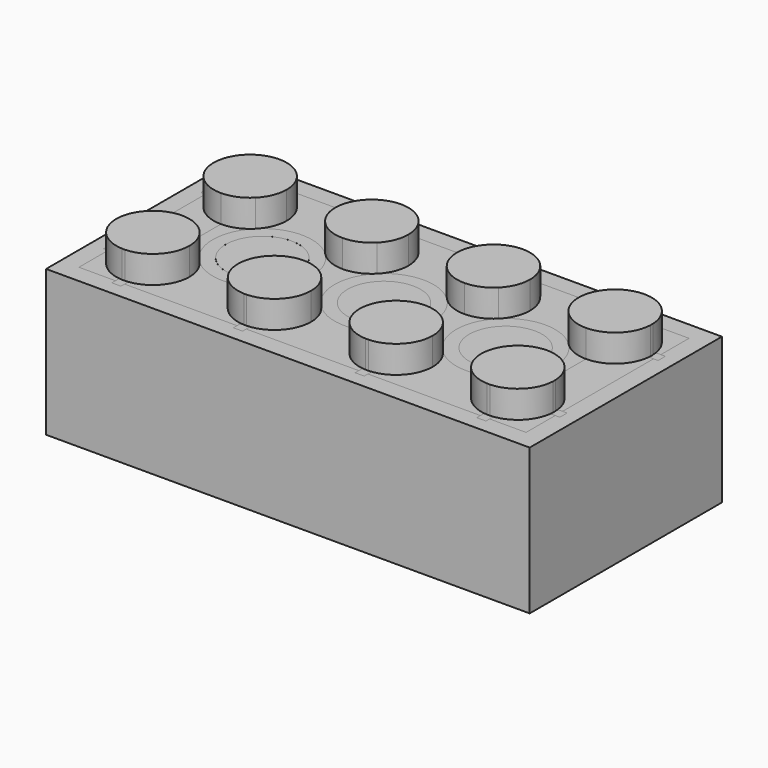
from build123d import *

# Parameters (mm, degrees)
F0_W     = 31.8
F0_H     = 15.8
F1_DEPTH = 9.6
F3_DEPTH = 1.8
F4_DEPTH = 9.6
F5_DEPTH = 1
F6_DEPTH = 1
F7_DEPTH = 1
F8_DEPTH = 1
F0_W_2   = 0.6
F0_H_2   = 0.3
F9_DEPTH = 9.6
F0_W_3   = 0.3
F0_H_3   = 0.6


# Not quite as in the source:
# - the program builds the solid bodies; features that only make, move or delete a surface that nothing else refers to are left out


with BuildPart() as f1:
    # F0 (on Top) → F1 (new body)
    with BuildSketch(Plane.XY):
        Rectangle(F0_W, F0_H)
        Polygon((-3.7, 6.7), (3.7, 6.7), (3.7, 7), (4.3, 7), (4.3, 6.7), (11.7, 6.7), (11.7, 7), (12.3, 7), (12.3, 6.7), (14.7, 6.7), (14.7, 4.3778601542), (15, 4.3778601542), (15, 3.7778601542), (14.7, 3.7778601542), (14.7, 0), (14.7, -3.7), (15, -3.7), (15, -4.3), (14.7, -4.3), (14.7, -6.7), (12.3, -6.7), (12.3, -7), (11.7, -7), (11.7, -6.7), (4.3, -6.7), (4.3, -7), (3.7, -7), (3.7, -6.7), (-3.7, -6.7), (-3.7, -7), (-4.3, -7), (-4.3, -6.7), (-11.7, -6.7), (-11.7, -7), (-12.3, -7), (-12.3, -6.7), (-14.7, -6.7), (-14.7, -4.3), (-15, -4.3), (-15, -3.7), (-14.7, -3.7), (-14.7, 0), (-14.7, 3.7), (-15, 3.7), (-15, 4.3), (-14.7, 4.3), (-14.7, 6.7), (-12.3, 6.7), (-12.3, 7), (-11.7, 7), (-11.7, 6.7), (-4.3, 6.7), (-4.3, 7), (-3.7, 7), align=None, mode=Mode.SUBTRACT)
    extrude(amount=-F1_DEPTH)


with BuildPart() as f3:
    # F0 (on Top) → F3 (new body)
    with BuildSketch(Plane.XY):
        with BuildLine():
            ThreePointArc((-14.4, 3.9056398611), (-13.6646718198, 2.2685926048), (-12, 1.5981457505))
            Line((-12, 1.5981457505), (-12, 2.7))
            ThreePointArc((-12, 2.7), (-12.9192388155, 4.9192388155), (-10.7, 4))
            Line((-10.7, 4), (-9.5981457505, 4))
            ThreePointArc((-9.5981457505, 4), (-10.2685926048, 5.6646718198), (-11.9056398611, 6.4))
            Line((-11.9056398611, 6.4), (-12.0943601389, 6.4))
            ThreePointArc((-12.0943601389, 6.4), (-13.6983674272, 5.6983674272), (-14.4, 4.0943601389))
            Line((-14.4, 4.0943601389), (-14.4, 3.9056398611))
        make_face()
        with BuildLine():
            ThreePointArc((-12, 1.5981457505), (-11.0808501792, 1.7809760157), (-10.3016325841, 2.3016325614))
            ThreePointArc((-10.3016325841, 2.3016325614), (-9.7809760219, 3.0808501643), (-9.5981457505, 4))
            Line((-9.5981457505, 4), (-10.7, 4))
            ThreePointArc((-10.7, 4), (-11.0807611845, 3.0807611845), (-12, 2.7))
            Line((-12, 2.7), (-12, 1.5981457505))
        make_face()
        with BuildLine():
            ThreePointArc((-10.7, 4), (-12.9192388155, 4.9192388155), (-12, 2.7))
            Line((-12, 2.7), (-12, 4))
            Line((-12, 4), (-10.7, 4))
        make_face()
        with BuildLine():
            Line((-12, 4), (-12, 2.7))
            ThreePointArc((-12, 2.7), (-11.0807611845, 3.0807611845), (-10.7, 4))
            Line((-10.7, 4), (-12, 4))
        make_face()
    extrude(amount=F3_DEPTH)


with BuildPart() as f3b:
    # F0 (on Top) → F3, piece 2 (new body)
    with BuildSketch(Plane.XY):
        with BuildLine():
            Line((-2.7, 4), (-1.5981457505, 4))
            ThreePointArc((-1.5981457505, 4), (-2.2685926048, 5.6646718198), (-3.9056398611, 6.4))
            Line((-3.9056398611, 6.4), (-4.0943601389, 6.4))
            ThreePointArc((-4.0943601389, 6.4), (-5.7314073952, 5.6646718198), (-6.4018542495, 4))
            Line((-6.4018542495, 4), (-5.3, 4))
            ThreePointArc((-5.3, 4), (-4, 5.3), (-2.7, 4))
        make_face()
        with BuildLine():
            ThreePointArc((-5.6983674332, 2.3016325788), (-4.9191498322, 1.7809760204), (-4, 1.5981457505))
            Line((-4, 1.5981457505), (-4, 2.7))
            ThreePointArc((-4, 2.7), (-4.9192388155, 3.0807611845), (-5.3, 4))
            Line((-5.3, 4), (-6.4018542495, 4))
            ThreePointArc((-6.4018542495, 4), (-6.2190239828, 3.0808501757), (-5.6983674332, 2.3016325788))
        make_face()
        with BuildLine():
            ThreePointArc((-4, 1.5981457505), (-3.0808501718, 1.7809760188), (-2.3016325728, 2.3016325728))
            ThreePointArc((-2.3016325728, 2.3016325728), (-1.7809760188, 3.0808501718), (-1.5981457505, 4))
            Line((-1.5981457505, 4), (-2.7, 4))
            ThreePointArc((-2.7, 4), (-3.0807611845, 3.0807611845), (-4, 2.7))
            Line((-4, 2.7), (-4, 1.5981457505))
        make_face()
        with BuildLine():
            Line((-4, 4), (-2.7, 4))
            ThreePointArc((-2.7, 4), (-4, 5.3), (-5.3, 4))
            Line((-5.3, 4), (-4, 4))
        make_face()
        with BuildLine():
            ThreePointArc((-5.3, 4), (-4.9192388155, 3.0807611845), (-4, 2.7))
            Line((-4, 2.7), (-4, 4))
            Line((-4, 4), (-5.3, 4))
        make_face()
        with BuildLine():
            Line((-4, 4), (-4, 2.7))
            ThreePointArc((-4, 2.7), (-3.0807611845, 3.0807611845), (-2.7, 4))
            Line((-2.7, 4), (-4, 4))
        make_face()
    extrude(amount=F3_DEPTH)


with BuildPart() as f3c:
    # F0 (on Top) → F3, piece 3 (new body)
    with BuildSketch(Plane.XY):
        with BuildLine():
            ThreePointArc((3.9056398611, 6.4), (2.2685926048, 5.6646718198), (1.5981457505, 4))
            Line((1.5981457505, 4), (2.7, 4))
            ThreePointArc((2.7, 4), (4, 5.3), (5.3, 4))
            Line((5.3, 4), (6.4018542495, 4))
            ThreePointArc((6.4018542495, 4), (5.7314073952, 5.6646718198), (4.0943601389, 6.4))
            Line((4.0943601389, 6.4), (3.9056398611, 6.4))
        make_face()
        with BuildLine():
            ThreePointArc((1.5981457505, 4), (1.7809760181, 3.0808501735), (2.3016325701, 2.3016325754))
            ThreePointArc((2.3016325701, 2.3016325754), (3.08085017, 1.7809760195), (4, 1.5981457505))
            Line((4, 1.5981457505), (4, 2.7))
            ThreePointArc((4, 2.7), (3.0807611845, 3.0807611845), (2.7, 4))
            Line((2.7, 4), (1.5981457505, 4))
        make_face()
        with BuildLine():
            Line((4, 2.7), (4, 1.5981457505))
            ThreePointArc((4, 1.5981457505), (4.9191498286, 1.780976019), (5.6983674279, 2.3016325734))
            ThreePointArc((5.6983674279, 2.3016325734), (6.2190239814, 3.0808501722), (6.4018542495, 4))
            Line((6.4018542495, 4), (5.3, 4))
            ThreePointArc((5.3, 4), (4.9192388155, 3.0807611845), (4, 2.7))
        make_face()
        with BuildLine():
            ThreePointArc((5.3, 4), (4, 5.3), (2.7, 4))
            Line((2.7, 4), (4, 4))
            Line((4, 4), (5.3, 4))
        make_face()
        with BuildLine():
            Line((4, 4), (2.7, 4))
            ThreePointArc((2.7, 4), (3.0807611845, 3.0807611845), (4, 2.7))
            Line((4, 2.7), (4, 4))
        make_face()
        with BuildLine():
            Line((4, 4), (4, 2.7))
            ThreePointArc((4, 2.7), (4.9192388155, 3.0807611845), (5.3, 4))
            Line((5.3, 4), (4, 4))
        make_face()
    extrude(amount=F3_DEPTH)


with BuildPart() as f3d:
    # F0 (on Top) → F3, piece 4 (new body)
    with BuildSketch(Plane.XY):
        with BuildLine():
            ThreePointArc((9.5981457505, 4), (9.7809760218, 3.0808501646), (10.3016325837, 2.3016325618))
            ThreePointArc((10.3016325837, 2.3016325618), (11.0808501789, 1.7809760159), (12, 1.5981457505))
            Line((12, 1.5981457505), (12, 2.7))
            ThreePointArc((12, 2.7), (11.0807611845, 3.0807611845), (10.7, 4))
            Line((10.7, 4), (9.5981457505, 4))
        make_face()
        with BuildLine():
            ThreePointArc((11.9056398611, 6.4), (10.2685926048, 5.6646718198), (9.5981457505, 4))
            Line((9.5981457505, 4), (10.7, 4))
            ThreePointArc((10.7, 4), (12, 5.3), (13.3, 4))
            ThreePointArc((13.3, 4), (12.9192388155, 3.0807611845), (12, 2.7))
            Line((12, 2.7), (12, 1.5981457505))
            ThreePointArc((12, 1.5981457505), (13.6646718198, 2.2685926048), (14.4, 3.9056398611))
            Line((14.4, 3.9056398611), (14.4, 4.0943601389))
            ThreePointArc((14.4, 4.0943601389), (13.6983674272, 5.6983674272), (12.0943601389, 6.4))
            Line((12.0943601389, 6.4), (11.9056398611, 6.4))
        make_face()
        with BuildLine():
            ThreePointArc((13.3, 4), (12, 5.3), (10.7, 4))
            Line((10.7, 4), (12, 4))
            Line((12, 4), (12, 2.7))
            ThreePointArc((12, 2.7), (12.9192388155, 3.0807611845), (13.3, 4))
        make_face()
        with BuildLine():
            Line((12, 4), (10.7, 4))
            ThreePointArc((10.7, 4), (11.0807611845, 3.0807611845), (12, 2.7))
            Line((12, 2.7), (12, 4))
        make_face()
    extrude(amount=F3_DEPTH)


with BuildPart() as f3e:
    # F0 (on Top) → F3, piece 5 (new body)
    with BuildSketch(Plane.XY):
        with BuildLine():
            ThreePointArc((12, -1.5981457505), (11.0808501718, -1.7809760188), (10.3016325728, -2.3016325728))
            ThreePointArc((10.3016325728, -2.3016325728), (9.7809760188, -3.0808501718), (9.5981457505, -4))
            Line((9.5981457505, -4), (10.7, -4))
            ThreePointArc((10.7, -4), (11.0807611845, -3.0807611845), (12, -2.7))
            Line((12, -2.7), (12, -1.5981457505))
        make_face()
        with BuildLine():
            ThreePointArc((14.4, -3.9056398611), (13.6646718198, -2.2685926048), (12, -1.5981457505))
            Line((12, -1.5981457505), (12, -2.7))
            ThreePointArc((12, -2.7), (12.9192388155, -3.0807611845), (13.3, -4))
            ThreePointArc((13.3, -4), (12, -5.3), (10.7, -4))
            Line((10.7, -4), (9.5981457505, -4))
            ThreePointArc((9.5981457505, -4), (10.2685926048, -5.6646718198), (11.9056398611, -6.4))
            Line((11.9056398611, -6.4), (12.0943601389, -6.4))
            ThreePointArc((12.0943601389, -6.4), (13.6983674272, -5.6983674272), (14.4, -4.0943601389))
            Line((14.4, -4.0943601389), (14.4, -3.9056398611))
        make_face()
        with BuildLine():
            Line((12, -4), (12, -2.7))
            ThreePointArc((12, -2.7), (11.0807611845, -3.0807611845), (10.7, -4))
            Line((10.7, -4), (12, -4))
        make_face()
        with BuildLine():
            ThreePointArc((13.3, -4), (12.9192388155, -3.0807611845), (12, -2.7))
            Line((12, -2.7), (12, -4))
            Line((12, -4), (10.7, -4))
            ThreePointArc((10.7, -4), (12, -5.3), (13.3, -4))
        make_face()
    extrude(amount=F3_DEPTH)


with BuildPart() as f3f:
    # F0 (on Top) → F3, piece 6 (new body)
    with BuildSketch(Plane.XY):
        with BuildLine():
            ThreePointArc((4, -1.5981457505), (3.0808501739, -1.7809760179), (2.3016325761, -2.3016325695))
            ThreePointArc((2.3016325761, -2.3016325695), (1.7809760197, -3.0808501696), (1.5981457505, -4))
            Line((1.5981457505, -4), (2.7, -4))
            ThreePointArc((2.7, -4), (3.0807611845, -3.0807611845), (4, -2.7))
            Line((4, -2.7), (4, -1.5981457505))
        make_face()
        with BuildLine():
            ThreePointArc((5.6983674292, -2.3016325747), (4.9191498295, -1.7809760193), (4, -1.5981457505))
            Line((4, -1.5981457505), (4, -2.7))
            ThreePointArc((4, -2.7), (4.9192388155, -3.0807611845), (5.3, -4))
            Line((5.3, -4), (6.4018542495, -4))
            ThreePointArc((6.4018542495, -4), (6.2190239817, -3.080850173), (5.6983674292, -2.3016325747))
        make_face()
        with BuildLine():
            Line((2.7, -4), (1.5981457505, -4))
            ThreePointArc((1.5981457505, -4), (2.2685926048, -5.6646718198), (3.9056398611, -6.4))
            Line((3.9056398611, -6.4), (4.0943601389, -6.4))
            ThreePointArc((4.0943601389, -6.4), (5.7314073952, -5.6646718198), (6.4018542495, -4))
            Line((6.4018542495, -4), (5.3, -4))
            ThreePointArc((5.3, -4), (4, -5.3), (2.7, -4))
        make_face()
        with BuildLine():
            ThreePointArc((5.3, -4), (4.9192388155, -3.0807611845), (4, -2.7))
            Line((4, -2.7), (4, -4))
            Line((4, -4), (5.3, -4))
        make_face()
        with BuildLine():
            Line((4, -4), (4, -2.7))
            ThreePointArc((4, -2.7), (3.0807611845, -3.0807611845), (2.7, -4))
            Line((2.7, -4), (4, -4))
        make_face()
        with BuildLine():
            Line((4, -4), (2.7, -4))
            ThreePointArc((2.7, -4), (4, -5.3), (5.3, -4))
            Line((5.3, -4), (4, -4))
        make_face()
    extrude(amount=F3_DEPTH)


with BuildPart() as f3g:
    # F0 (on Top) → F3, piece 7 (new body)
    with BuildSketch(Plane.XY):
        with BuildLine():
            ThreePointArc((-1.5981457505, -4), (-1.7809760197, -3.0808501696), (-2.3016325761, -2.3016325695))
            ThreePointArc((-2.3016325761, -2.3016325695), (-3.0808501739, -1.7809760179), (-4, -1.5981457505))
            Line((-4, -1.5981457505), (-4, -2.7))
            ThreePointArc((-4, -2.7), (-3.0807611845, -3.0807611845), (-2.7, -4))
            Line((-2.7, -4), (-1.5981457505, -4))
        make_face()
        with BuildLine():
            Line((-4, -2.7), (-4, -1.5981457505))
            ThreePointArc((-4, -1.5981457505), (-4.9191498282, -1.7809760188), (-5.6983674272, -2.3016325728))
            ThreePointArc((-5.6983674272, -2.3016325728), (-6.2190239812, -3.0808501718), (-6.4018542495, -4))
            Line((-6.4018542495, -4), (-5.3, -4))
            ThreePointArc((-5.3, -4), (-4.9192388155, -3.0807611845), (-4, -2.7))
        make_face()
        with BuildLine():
            ThreePointArc((-3.9056398611, -6.4), (-2.2685926048, -5.6646718198), (-1.5981457505, -4))
            Line((-1.5981457505, -4), (-2.7, -4))
            ThreePointArc((-2.7, -4), (-4, -5.3), (-5.3, -4))
            Line((-5.3, -4), (-6.4018542495, -4))
            ThreePointArc((-6.4018542495, -4), (-5.7314073952, -5.6646718198), (-4.0943601389, -6.4))
            Line((-4.0943601389, -6.4), (-3.9056398611, -6.4))
        make_face()
        with BuildLine():
            Line((-4, -4), (-2.7, -4))
            ThreePointArc((-2.7, -4), (-3.0807611845, -3.0807611845), (-4, -2.7))
            Line((-4, -2.7), (-4, -4))
        make_face()
        with BuildLine():
            Line((-4, -4), (-4, -2.7))
            ThreePointArc((-4, -2.7), (-4.9192388155, -3.0807611845), (-5.3, -4))
            Line((-5.3, -4), (-4, -4))
        make_face()
        with BuildLine():
            ThreePointArc((-5.3, -4), (-4, -5.3), (-2.7, -4))
            Line((-2.7, -4), (-4, -4))
            Line((-4, -4), (-5.3, -4))
        make_face()
    extrude(amount=F3_DEPTH)


with BuildPart() as f3h:
    # F0 (on Top) → F3, piece 8 (new body)
    with BuildSketch(Plane.XY):
        with BuildLine():
            ThreePointArc((-11.9056398611, -6.4), (-10.2685926048, -5.6646718198), (-9.5981457505, -4))
            Line((-9.5981457505, -4), (-10.7, -4))
            ThreePointArc((-10.7, -4), (-12.9192388155, -4.9192388155), (-12, -2.7))
            Line((-12, -2.7), (-12, -1.5981457505))
            ThreePointArc((-12, -1.5981457505), (-13.6646718198, -2.2685926048), (-14.4, -3.9056398611))
            Line((-14.4, -3.9056398611), (-14.4, -4.0943601389))
            ThreePointArc((-14.4, -4.0943601389), (-13.6983674272, -5.6983674272), (-12.0943601389, -6.4))
            Line((-12.0943601389, -6.4), (-11.9056398611, -6.4))
        make_face()
        with BuildLine():
            ThreePointArc((-9.5981457505, -4), (-9.7809760188, -3.0808501718), (-10.3016325728, -2.3016325728))
            ThreePointArc((-10.3016325728, -2.3016325728), (-11.0808501718, -1.7809760188), (-12, -1.5981457505))
            Line((-12, -1.5981457505), (-12, -2.7))
            ThreePointArc((-12, -2.7), (-11.0807611845, -3.0807611845), (-10.7, -4))
            Line((-10.7, -4), (-9.5981457505, -4))
        make_face()
        with BuildLine():
            Line((-12, -4), (-10.7, -4))
            ThreePointArc((-10.7, -4), (-11.0807611845, -3.0807611845), (-12, -2.7))
            Line((-12, -2.7), (-12, -4))
        make_face()
        with BuildLine():
            ThreePointArc((-12, -2.7), (-12.9192388155, -4.9192388155), (-10.7, -4))
            Line((-10.7, -4), (-12, -4))
            Line((-12, -4), (-12, -2.7))
        make_face()
    extrude(amount=F3_DEPTH)


with BuildPart() as f4:
    # F0 (on Top) → F4 (new body)
    with BuildSketch(Plane.XY):
        with BuildLine():
            ThreePointArc((-10.3016325728, -2.3016325728), (-8, -3.255), (-5.6983674272, -2.3016325728))
            ThreePointArc((-5.6983674272, -2.3016325728), (-4.9927721217, -1.2456345723), (-4.745, 0))
            Line((-4.745, 0), (-5.6, 0))
            ThreePointArc((-5.6, 0), (-8, -2.4), (-10.4, 0))
            Line((-10.4, 0), (-11.255, 0))
            ThreePointArc((-11.255, 0), (-11.0072278783, -1.2456345723), (-10.3016325728, -2.3016325728))
        make_face()
        with BuildLine():
            ThreePointArc((-4.745, 0), (-4.9927721233, 1.2456345763), (-5.6983674332, 2.3016325788))
            ThreePointArc((-5.6983674332, 2.3016325788), (-8.0000000123, 3.255), (-10.3016325841, 2.3016325614))
            ThreePointArc((-10.3016325841, 2.3016325614), (-11.0072278814, 1.2456345649), (-11.255, 0))
            Line((-11.255, 0), (-10.4, 0))
            ThreePointArc((-10.4, 0), (-8, 2.4), (-5.6, 0))
            Line((-5.6, 0), (-4.745, 0))
        make_face()
    extrude(amount=-F4_DEPTH)


with BuildPart() as f4b:
    # F0 (on Top) → F4, piece 2 (new body)
    with BuildSketch(Plane.XY):
        with BuildLine():
            ThreePointArc((2.3016325761, -2.3016325695), (3.0072278792, -1.2456345702), (3.255, 0))
            Line((3.255, 0), (2.4, 0))
            ThreePointArc((2.4, 0), (0, -2.4), (-2.4, 0))
            Line((-2.4, 0), (-3.255, 0))
            ThreePointArc((-3.255, 0), (-3.0072278792, -1.2456345702), (-2.3016325761, -2.3016325695))
            ThreePointArc((-2.3016325761, -2.3016325695), (0, -3.255), (2.3016325761, -2.3016325695))
        make_face()
        with BuildLine():
            Line((2.4, 0), (3.255, 0))
            ThreePointArc((3.255, 0), (3.0072278776, 1.2456345741), (2.3016325701, 2.3016325754))
            ThreePointArc((2.3016325701, 2.3016325754), (-1.9e-09, 3.255), (-2.3016325728, 2.3016325728))
            ThreePointArc((-2.3016325728, 2.3016325728), (-3.0072278783, 1.2456345723), (-3.255, 0))
            Line((-3.255, 0), (-2.4, 0))
            ThreePointArc((-2.4, 0), (0, 2.4), (2.4, 0))
        make_face()
    extrude(amount=-F4_DEPTH)


with BuildPart() as f4c:
    # F0 (on Top) → F4, piece 3 (new body)
    with BuildSketch(Plane.XY):
        with BuildLine():
            Line((5.6, 0), (4.745, 0))
            ThreePointArc((4.745, 0), (4.9927721222, -1.2456345736), (5.6983674292, -2.3016325747))
            ThreePointArc((5.6983674292, -2.3016325747), (8.0000000014, -3.255), (10.3016325728, -2.3016325728))
            ThreePointArc((10.3016325728, -2.3016325728), (11.0072278783, -1.2456345723), (11.255, 0))
            Line((11.255, 0), (10.4, 0))
            ThreePointArc((10.4, 0), (8, -2.4), (5.6, 0))
        make_face()
        with BuildLine():
            ThreePointArc((5.6983674279, 2.3016325734), (4.9927721218, 1.2456345728), (4.745, 0))
            Line((4.745, 0), (5.6, 0))
            ThreePointArc((5.6, 0), (8, 2.4), (10.4, 0))
            Line((10.4, 0), (11.255, 0))
            ThreePointArc((11.255, 0), (11.0072278813, 1.2456345652), (10.3016325837, 2.3016325618))
            ThreePointArc((10.3016325837, 2.3016325618), (8.0000000082, 3.255), (5.6983674279, 2.3016325734))
        make_face()
    extrude(amount=-F4_DEPTH)


with BuildPart() as f5:
    # F0 (on Top) → F5 (new body)
    with BuildSketch(Plane.XY):
        with BuildLine():
            Line((12.3, 6.4), (12.0943601389, 6.4))
            ThreePointArc((12.0943601389, 6.4), (13.6983674272, 5.6983674272), (14.4, 4.0943601389))
            Line((14.4, 4.0943601389), (14.4, 4.3778601542))
            Line((14.4, 4.3778601542), (14.7, 4.3778601542))
            Line((14.7, 4.3778601542), (14.7, 6.7))
            Line((14.7, 6.7), (12.3, 6.7))
            Line((12.3, 6.7), (12.3, 6.4))
        make_face()
        with BuildLine():
            Line((11.7, 6.4), (11.9056398611, 6.4))
            ThreePointArc((11.9056398611, 6.4), (12, 6.4018542495), (12.0943601389, 6.4))
            Line((12.0943601389, 6.4), (12.3, 6.4))
            Line((12.3, 6.4), (12.3, 6.7))
            Line((12.3, 6.7), (11.7, 6.7))
            Line((11.7, 6.7), (11.7, 6.4))
        make_face()
        with BuildLine():
            Line((4.3, 6.4), (4.0943601389, 6.4))
            ThreePointArc((4.0943601389, 6.4), (5.7314073952, 5.6646718198), (6.4018542495, 4))
            Line((6.4018542495, 4), (9.5981457505, 4))
            ThreePointArc((9.5981457505, 4), (10.2685926048, 5.6646718198), (11.9056398611, 6.4))
            Line((11.9056398611, 6.4), (11.7, 6.4))
            Line((11.7, 6.4), (11.7, 6.7))
            Line((11.7, 6.7), (4.3, 6.7))
            Line((4.3, 6.7), (4.3, 6.4))
        make_face()
        with BuildLine():
            Line((3.7, 6.4), (3.9056398611, 6.4))
            ThreePointArc((3.9056398611, 6.4), (4, 6.4018542495), (4.0943601389, 6.4))
            Line((4.0943601389, 6.4), (4.3, 6.4))
            Line((4.3, 6.4), (4.3, 6.7))
            Line((4.3, 6.7), (3.7, 6.7))
            Line((3.7, 6.7), (3.7, 6.4))
        make_face()
        with BuildLine():
            Line((-1.5981457505, 4), (1.5981457505, 4))
            ThreePointArc((1.5981457505, 4), (2.2685926048, 5.6646718198), (3.9056398611, 6.4))
            Line((3.9056398611, 6.4), (3.7, 6.4))
            Line((3.7, 6.4), (3.7, 6.7))
            Line((3.7, 6.7), (-3.7, 6.7))
            Line((-3.7, 6.7), (-3.7, 6.4))
            Line((-3.7, 6.4), (-3.9056398611, 6.4))
            ThreePointArc((-3.9056398611, 6.4), (-2.2685926048, 5.6646718198), (-1.5981457505, 4))
        make_face()
        with BuildLine():
            ThreePointArc((-4.0943601389, 6.4), (-4, 6.4018542495), (-3.9056398611, 6.4))
            Line((-3.9056398611, 6.4), (-3.7, 6.4))
            Line((-3.7, 6.4), (-3.7, 6.7))
            Line((-3.7, 6.7), (-4.3, 6.7))
            Line((-4.3, 6.7), (-4.3, 6.4))
            Line((-4.3, 6.4), (-4.0943601389, 6.4))
        make_face()
        with BuildLine():
            Line((-9.5981457505, 4), (-6.4018542495, 4))
            ThreePointArc((-6.4018542495, 4), (-5.7314073952, 5.6646718198), (-4.0943601389, 6.4))
            Line((-4.0943601389, 6.4), (-4.3, 6.4))
            Line((-4.3, 6.4), (-4.3, 6.7))
            Line((-4.3, 6.7), (-11.7, 6.7))
            Line((-11.7, 6.7), (-11.7, 6.4))
            Line((-11.7, 6.4), (-11.9056398611, 6.4))
            ThreePointArc((-11.9056398611, 6.4), (-10.2685926048, 5.6646718198), (-9.5981457505, 4))
        make_face()
        with BuildLine():
            ThreePointArc((-12.0943601389, 6.4), (-12, 6.4018542495), (-11.9056398611, 6.4))
            Line((-11.9056398611, 6.4), (-11.7, 6.4))
            Line((-11.7, 6.4), (-11.7, 6.7))
            Line((-11.7, 6.7), (-12.3, 6.7))
            Line((-12.3, 6.7), (-12.3, 6.4))
            Line((-12.3, 6.4), (-12.0943601389, 6.4))
        make_face()
        with BuildLine():
            Line((-14.4, 4.3), (-14.4, 4.0943601389))
            ThreePointArc((-14.4, 4.0943601389), (-13.6983674272, 5.6983674272), (-12.0943601389, 6.4))
            Line((-12.0943601389, 6.4), (-12.3, 6.4))
            Line((-12.3, 6.4), (-12.3, 6.7))
            Line((-12.3, 6.7), (-14.7, 6.7))
            Line((-14.7, 6.7), (-14.7, 4.3))
            Line((-14.7, 4.3), (-14.4, 4.3))
        make_face()
        with BuildLine():
            ThreePointArc((6.4018542495, 4), (6.2190239814, 3.0808501722), (5.6983674279, 2.3016325734))
            ThreePointArc((5.6983674279, 2.3016325734), (8.0000000082, 3.255), (10.3016325837, 2.3016325618))
            ThreePointArc((10.3016325837, 2.3016325618), (9.7809760218, 3.0808501646), (9.5981457505, 4))
            Line((9.5981457505, 4), (6.4018542495, 4))
        make_face()
        with BuildLine():
            ThreePointArc((-2.3016325728, 2.3016325728), (-1.9e-09, 3.255), (2.3016325701, 2.3016325754))
            ThreePointArc((2.3016325701, 2.3016325754), (1.7809760181, 3.0808501735), (1.5981457505, 4))
            Line((1.5981457505, 4), (-1.5981457505, 4))
            ThreePointArc((-1.5981457505, 4), (-1.7809760188, 3.0808501718), (-2.3016325728, 2.3016325728))
        make_face()
        with BuildLine():
            ThreePointArc((-10.3016325841, 2.3016325614), (-8.0000000123, 3.255), (-5.6983674332, 2.3016325788))
            ThreePointArc((-5.6983674332, 2.3016325788), (-6.2190239828, 3.0808501757), (-6.4018542495, 4))
            Line((-6.4018542495, 4), (-9.5981457505, 4))
            ThreePointArc((-9.5981457505, 4), (-9.7809760219, 3.0808501643), (-10.3016325841, 2.3016325614))
        make_face()
    extrude(amount=-F5_DEPTH)


with BuildPart() as f5b:
    # F0 (on Top) → F5, piece 2 (new body)
    with BuildSketch(Plane.XY):
        with BuildLine():
            Line((14.4, -4.3), (14.4, -4.0943601389))
            ThreePointArc((14.4, -4.0943601389), (13.6983674272, -5.6983674272), (12.0943601389, -6.4))
            Line((12.0943601389, -6.4), (12.3, -6.4))
            Line((12.3, -6.4), (12.3, -6.7))
            Line((12.3, -6.7), (14.7, -6.7))
            Line((14.7, -6.7), (14.7, -4.3))
            Line((14.7, -4.3), (14.4, -4.3))
        make_face()
        with BuildLine():
            ThreePointArc((12.0943601389, -6.4), (12, -6.4018542495), (11.9056398611, -6.4))
            Line((11.9056398611, -6.4), (11.7, -6.4))
            Line((11.7, -6.4), (11.7, -6.7))
            Line((11.7, -6.7), (12.3, -6.7))
            Line((12.3, -6.7), (12.3, -6.4))
            Line((12.3, -6.4), (12.0943601389, -6.4))
        make_face()
        with BuildLine():
            Line((9.5981457505, -4), (6.4018542495, -4))
            ThreePointArc((6.4018542495, -4), (5.7314073952, -5.6646718198), (4.0943601389, -6.4))
            Line((4.0943601389, -6.4), (4.3, -6.4))
            Line((4.3, -6.4), (4.3, -6.7))
            Line((4.3, -6.7), (11.7, -6.7))
            Line((11.7, -6.7), (11.7, -6.4))
            Line((11.7, -6.4), (11.9056398611, -6.4))
            ThreePointArc((11.9056398611, -6.4), (10.2685926048, -5.6646718198), (9.5981457505, -4))
        make_face()
        with BuildLine():
            ThreePointArc((4.0943601389, -6.4), (4, -6.4018542495), (3.9056398611, -6.4))
            Line((3.9056398611, -6.4), (3.7, -6.4))
            Line((3.7, -6.4), (3.7, -6.7))
            Line((3.7, -6.7), (4.3, -6.7))
            Line((4.3, -6.7), (4.3, -6.4))
            Line((4.3, -6.4), (4.0943601389, -6.4))
        make_face()
        with BuildLine():
            ThreePointArc((3.9056398611, -6.4), (2.2685926048, -5.6646718198), (1.5981457505, -4))
            Line((1.5981457505, -4), (-1.5981457505, -4))
            ThreePointArc((-1.5981457505, -4), (-2.2685926048, -5.6646718198), (-3.9056398611, -6.4))
            Line((-3.9056398611, -6.4), (-3.7, -6.4))
            Line((-3.7, -6.4), (-3.7, -6.7))
            Line((-3.7, -6.7), (3.7, -6.7))
            Line((3.7, -6.7), (3.7, -6.4))
            Line((3.7, -6.4), (3.9056398611, -6.4))
        make_face()
        with BuildLine():
            Line((-3.7, -6.4), (-3.9056398611, -6.4))
            ThreePointArc((-3.9056398611, -6.4), (-4, -6.4018542495), (-4.0943601389, -6.4))
            Line((-4.0943601389, -6.4), (-4.3, -6.4))
            Line((-4.3, -6.4), (-4.3, -6.7))
            Line((-4.3, -6.7), (-3.7, -6.7))
            Line((-3.7, -6.7), (-3.7, -6.4))
        make_face()
        with BuildLine():
            Line((-4.3, -6.4), (-4.0943601389, -6.4))
            ThreePointArc((-4.0943601389, -6.4), (-5.7314073952, -5.6646718198), (-6.4018542495, -4))
            Line((-6.4018542495, -4), (-9.5981457505, -4))
            ThreePointArc((-9.5981457505, -4), (-10.2685926048, -5.6646718198), (-11.9056398611, -6.4))
            Line((-11.9056398611, -6.4), (-11.7, -6.4))
            Line((-11.7, -6.4), (-11.7, -6.7))
            Line((-11.7, -6.7), (-4.3, -6.7))
            Line((-4.3, -6.7), (-4.3, -6.4))
        make_face()
        with BuildLine():
            Line((-11.7, -6.4), (-11.9056398611, -6.4))
            ThreePointArc((-11.9056398611, -6.4), (-12, -6.4018542495), (-12.0943601389, -6.4))
            Line((-12.0943601389, -6.4), (-12.3, -6.4))
            Line((-12.3, -6.4), (-12.3, -6.7))
            Line((-12.3, -6.7), (-11.7, -6.7))
            Line((-11.7, -6.7), (-11.7, -6.4))
        make_face()
        with BuildLine():
            Line((-12.3, -6.4), (-12.0943601389, -6.4))
            ThreePointArc((-12.0943601389, -6.4), (-13.6983674272, -5.6983674272), (-14.4, -4.0943601389))
            Line((-14.4, -4.0943601389), (-14.4, -4.3))
            Line((-14.4, -4.3), (-14.7, -4.3))
            Line((-14.7, -4.3), (-14.7, -6.7))
            Line((-14.7, -6.7), (-12.3, -6.7))
            Line((-12.3, -6.7), (-12.3, -6.4))
        make_face()
        with BuildLine():
            ThreePointArc((10.3016325728, -2.3016325728), (8.0000000014, -3.255), (5.6983674292, -2.3016325747))
            ThreePointArc((5.6983674292, -2.3016325747), (6.2190239817, -3.080850173), (6.4018542495, -4))
            Line((6.4018542495, -4), (9.5981457505, -4))
            ThreePointArc((9.5981457505, -4), (9.7809760188, -3.0808501718), (10.3016325728, -2.3016325728))
        make_face()
        with BuildLine():
            ThreePointArc((1.5981457505, -4), (1.7809760197, -3.0808501696), (2.3016325761, -2.3016325695))
            ThreePointArc((2.3016325761, -2.3016325695), (0, -3.255), (-2.3016325761, -2.3016325695))
            ThreePointArc((-2.3016325761, -2.3016325695), (-1.7809760197, -3.0808501696), (-1.5981457505, -4))
            Line((-1.5981457505, -4), (1.5981457505, -4))
        make_face()
        with BuildLine():
            ThreePointArc((-6.4018542495, -4), (-6.2190239812, -3.0808501718), (-5.6983674272, -2.3016325728))
            ThreePointArc((-5.6983674272, -2.3016325728), (-8, -3.255), (-10.3016325728, -2.3016325728))
            ThreePointArc((-10.3016325728, -2.3016325728), (-9.7809760188, -3.0808501718), (-9.5981457505, -4))
            Line((-9.5981457505, -4), (-6.4018542495, -4))
        make_face()
    extrude(amount=-F5_DEPTH)


with BuildPart() as f5c:
    # F0 (on Top) → F5, piece 3 (new body)
    with BuildSketch(Plane.XY):
        with BuildLine():
            Line((-12, 0), (-12, 1.5981457505))
            ThreePointArc((-12, 1.5981457505), (-13.6646718198, 2.2685926048), (-14.4, 3.9056398611))
            Line((-14.4, 3.9056398611), (-14.4, 3.7))
            Line((-14.4, 3.7), (-14.7, 3.7))
            Line((-14.7, 3.7), (-14.7, 0))
            Line((-14.7, 0), (-12, 0))
        make_face()
        with BuildLine():
            ThreePointArc((-14.4, -3.9056398611), (-13.6646718198, -2.2685926048), (-12, -1.5981457505))
            Line((-12, -1.5981457505), (-12, 0))
            Line((-12, 0), (-14.7, 0))
            Line((-14.7, 0), (-14.7, -3.7))
            Line((-14.7, -3.7), (-14.4, -3.7))
            Line((-14.4, -3.7), (-14.4, -3.9056398611))
        make_face()
    extrude(amount=-F5_DEPTH)


with BuildPart() as f5d:
    # F0 (on Top) → F5, piece 4 (new body)
    with BuildSketch(Plane.XY):
        with BuildLine():
            ThreePointArc((14.4, 3.9056398611), (13.6646718198, 2.2685926048), (12, 1.5981457505))
            Line((12, 1.5981457505), (12, 0))
            Line((12, 0), (14.7, 0))
            Line((14.7, 0), (14.7, 3.7778601542))
            Line((14.7, 3.7778601542), (14.4, 3.7778601542))
            Line((14.4, 3.7778601542), (14.4, 3.9056398611))
        make_face()
        with BuildLine():
            Line((12, 0), (12, -1.5981457505))
            ThreePointArc((12, -1.5981457505), (13.6646718198, -2.2685926048), (14.4, -3.9056398611))
            Line((14.4, -3.9056398611), (14.4, -3.7))
            Line((14.4, -3.7), (14.7, -3.7))
            Line((14.7, -3.7), (14.7, 0))
            Line((14.7, 0), (12, 0))
        make_face()
    extrude(amount=-F5_DEPTH)


with BuildPart() as f6:
    # F0 (on Top) → F6 (new body)
    with BuildSketch(Plane.XY):
        with BuildLine():
            ThreePointArc((-10.4, 0), (-8, -2.4), (-5.6, 0))
            Line((-5.6, 0), (-8, 0))
            Line((-8, 0), (-10.4, 0))
        make_face()
        with BuildLine():
            Line((-8, 0), (-5.6, 0))
            ThreePointArc((-5.6, 0), (-8, 2.4), (-10.4, 0))
            Line((-10.4, 0), (-8, 0))
        make_face()
    extrude(amount=-F6_DEPTH)


with BuildPart() as f6b:
    # F0 (on Top) → F6, piece 2 (new body)
    with BuildSketch(Plane.XY):
        with BuildLine():
            Line((0, 0), (2.4, 0))
            ThreePointArc((2.4, 0), (0, 2.4), (-2.4, 0))
            Line((-2.4, 0), (0, 0))
        make_face()
        with BuildLine():
            ThreePointArc((-2.4, 0), (0, -2.4), (2.4, 0))
            Line((2.4, 0), (0, 0))
            Line((0, 0), (-2.4, 0))
        make_face()
    extrude(amount=-F6_DEPTH)


with BuildPart() as f6c:
    # F0 (on Top) → F6, piece 3 (new body)
    with BuildSketch(Plane.XY):
        with BuildLine():
            ThreePointArc((10.4, 0), (8, 2.4), (5.6, 0))
            Line((5.6, 0), (8, 0))
            Line((8, 0), (10.4, 0))
        make_face()
        with BuildLine():
            Line((8, 0), (5.6, 0))
            ThreePointArc((5.6, 0), (8, -2.4), (10.4, 0))
            Line((10.4, 0), (8, 0))
        make_face()
    extrude(amount=-F6_DEPTH)


with BuildPart() as f7:
    # F0 (on Top) → F7 (new body)
    with BuildSketch(Plane.XY):
        with BuildLine():
            ThreePointArc((-11.255, 0), (-11.0072278814, 1.2456345649), (-10.3016325841, 2.3016325614))
            ThreePointArc((-10.3016325841, 2.3016325614), (-11.0808501792, 1.7809760157), (-12, 1.5981457505))
            Line((-12, 1.5981457505), (-12, 0))
            Line((-12, 0), (-11.255, 0))
        make_face()
        with BuildLine():
            ThreePointArc((-12, -1.5981457505), (-11.0808501718, -1.7809760188), (-10.3016325728, -2.3016325728))
            ThreePointArc((-10.3016325728, -2.3016325728), (-11.0072278783, -1.2456345723), (-11.255, 0))
            Line((-11.255, 0), (-12, 0))
            Line((-12, 0), (-12, -1.5981457505))
        make_face()
    extrude(amount=-F7_DEPTH)


with BuildPart() as f7b:
    # F0 (on Top) → F7, piece 2 (new body)
    with BuildSketch(Plane.XY):
        with BuildLine():
            ThreePointArc((-5.6983674272, -2.3016325728), (-4.9191498282, -1.7809760188), (-4, -1.5981457505))
            Line((-4, -1.5981457505), (-4, 0))
            Line((-4, 0), (-4.745, 0))
            ThreePointArc((-4.745, 0), (-4.9927721217, -1.2456345723), (-5.6983674272, -2.3016325728))
        make_face()
        with BuildLine():
            Line((-4, 0), (-4, 1.5981457505))
            ThreePointArc((-4, 1.5981457505), (-4.9191498322, 1.7809760204), (-5.6983674332, 2.3016325788))
            ThreePointArc((-5.6983674332, 2.3016325788), (-4.9927721233, 1.2456345763), (-4.745, 0))
            Line((-4.745, 0), (-4, 0))
        make_face()
        with BuildLine():
            ThreePointArc((-3.255, 0), (-3.0072278783, 1.2456345723), (-2.3016325728, 2.3016325728))
            ThreePointArc((-2.3016325728, 2.3016325728), (-3.0808501718, 1.7809760188), (-4, 1.5981457505))
            Line((-4, 1.5981457505), (-4, 0))
            Line((-4, 0), (-3.255, 0))
        make_face()
        with BuildLine():
            ThreePointArc((-4, -1.5981457505), (-3.0808501739, -1.7809760179), (-2.3016325761, -2.3016325695))
            ThreePointArc((-2.3016325761, -2.3016325695), (-3.0072278792, -1.2456345702), (-3.255, 0))
            Line((-3.255, 0), (-4, 0))
            Line((-4, 0), (-4, -1.5981457505))
        make_face()
    extrude(amount=-F7_DEPTH)


with BuildPart() as f7c:
    # F0 (on Top) → F7, piece 3 (new body)
    with BuildSketch(Plane.XY):
        with BuildLine():
            ThreePointArc((2.3016325701, 2.3016325754), (3.0072278776, 1.2456345741), (3.255, 0))
            Line((3.255, 0), (4, 0))
            Line((4, 0), (4, 1.5981457505))
            ThreePointArc((4, 1.5981457505), (3.08085017, 1.7809760195), (2.3016325701, 2.3016325754))
        make_face()
        with BuildLine():
            Line((4, 1.5981457505), (4, 0))
            Line((4, 0), (4.745, 0))
            ThreePointArc((4.745, 0), (4.9927721218, 1.2456345728), (5.6983674279, 2.3016325734))
            ThreePointArc((5.6983674279, 2.3016325734), (4.9191498286, 1.780976019), (4, 1.5981457505))
        make_face()
        with BuildLine():
            Line((4.745, 0), (4, 0))
            Line((4, 0), (4, -1.5981457505))
            ThreePointArc((4, -1.5981457505), (4.9191498295, -1.7809760193), (5.6983674292, -2.3016325747))
            ThreePointArc((5.6983674292, -2.3016325747), (4.9927721222, -1.2456345736), (4.745, 0))
        make_face()
        with BuildLine():
            Line((4, 0), (3.255, 0))
            ThreePointArc((3.255, 0), (3.0072278792, -1.2456345702), (2.3016325761, -2.3016325695))
            ThreePointArc((2.3016325761, -2.3016325695), (3.0808501739, -1.7809760179), (4, -1.5981457505))
            Line((4, -1.5981457505), (4, 0))
        make_face()
    extrude(amount=-F7_DEPTH)


with BuildPart() as f7d:
    # F0 (on Top) → F7, piece 4 (new body)
    with BuildSketch(Plane.XY):
        with BuildLine():
            ThreePointArc((12, 1.5981457505), (11.0808501789, 1.7809760159), (10.3016325837, 2.3016325618))
            ThreePointArc((10.3016325837, 2.3016325618), (11.0072278813, 1.2456345652), (11.255, 0))
            Line((11.255, 0), (12, 0))
            Line((12, 0), (12, 1.5981457505))
        make_face()
        with BuildLine():
            ThreePointArc((11.255, 0), (11.0072278783, -1.2456345723), (10.3016325728, -2.3016325728))
            ThreePointArc((10.3016325728, -2.3016325728), (11.0808501718, -1.7809760188), (12, -1.5981457505))
            Line((12, -1.5981457505), (12, 0))
            Line((12, 0), (11.255, 0))
        make_face()
    extrude(amount=-F7_DEPTH)


with BuildPart() as f8:
    # F0 (on Top) → F8 (new body)
    with BuildSketch(Plane.XY):
        with BuildLine():
            ThreePointArc((-11.9056398611, -6.4), (-10.2685926048, -5.6646718198), (-9.5981457505, -4))
            Line((-9.5981457505, -4), (-10.7, -4))
            ThreePointArc((-10.7, -4), (-12.9192388155, -4.9192388155), (-12, -2.7))
            Line((-12, -2.7), (-12, -1.5981457505))
            ThreePointArc((-12, -1.5981457505), (-13.6646718198, -2.2685926048), (-14.4, -3.9056398611))
            Line((-14.4, -3.9056398611), (-14.4, -4.0943601389))
            ThreePointArc((-14.4, -4.0943601389), (-13.6983674272, -5.6983674272), (-12.0943601389, -6.4))
            Line((-12.0943601389, -6.4), (-11.9056398611, -6.4))
        make_face()
        with BuildLine():
            ThreePointArc((-9.5981457505, -4), (-9.7809760188, -3.0808501718), (-10.3016325728, -2.3016325728))
            ThreePointArc((-10.3016325728, -2.3016325728), (-11.0808501718, -1.7809760188), (-12, -1.5981457505))
            Line((-12, -1.5981457505), (-12, -2.7))
            ThreePointArc((-12, -2.7), (-11.0807611845, -3.0807611845), (-10.7, -4))
            Line((-10.7, -4), (-9.5981457505, -4))
        make_face()
    extrude(amount=-F8_DEPTH)


with BuildPart() as f8b:
    # F0 (on Top) → F8, piece 2 (new body)
    with BuildSketch(Plane.XY):
        with BuildLine():
            ThreePointArc((-3.9056398611, -6.4), (-2.2685926048, -5.6646718198), (-1.5981457505, -4))
            Line((-1.5981457505, -4), (-2.7, -4))
            ThreePointArc((-2.7, -4), (-4, -5.3), (-5.3, -4))
            Line((-5.3, -4), (-6.4018542495, -4))
            ThreePointArc((-6.4018542495, -4), (-5.7314073952, -5.6646718198), (-4.0943601389, -6.4))
            Line((-4.0943601389, -6.4), (-3.9056398611, -6.4))
        make_face()
        with BuildLine():
            Line((-4, -2.7), (-4, -1.5981457505))
            ThreePointArc((-4, -1.5981457505), (-4.9191498282, -1.7809760188), (-5.6983674272, -2.3016325728))
            ThreePointArc((-5.6983674272, -2.3016325728), (-6.2190239812, -3.0808501718), (-6.4018542495, -4))
            Line((-6.4018542495, -4), (-5.3, -4))
            ThreePointArc((-5.3, -4), (-4.9192388155, -3.0807611845), (-4, -2.7))
        make_face()
        with BuildLine():
            ThreePointArc((-1.5981457505, -4), (-1.7809760197, -3.0808501696), (-2.3016325761, -2.3016325695))
            ThreePointArc((-2.3016325761, -2.3016325695), (-3.0808501739, -1.7809760179), (-4, -1.5981457505))
            Line((-4, -1.5981457505), (-4, -2.7))
            ThreePointArc((-4, -2.7), (-3.0807611845, -3.0807611845), (-2.7, -4))
            Line((-2.7, -4), (-1.5981457505, -4))
        make_face()
    extrude(amount=-F8_DEPTH)


with BuildPart() as f8c:
    # F0 (on Top) → F8, piece 3 (new body)
    with BuildSketch(Plane.XY):
        with BuildLine():
            Line((2.7, -4), (1.5981457505, -4))
            ThreePointArc((1.5981457505, -4), (2.2685926048, -5.6646718198), (3.9056398611, -6.4))
            Line((3.9056398611, -6.4), (4.0943601389, -6.4))
            ThreePointArc((4.0943601389, -6.4), (5.7314073952, -5.6646718198), (6.4018542495, -4))
            Line((6.4018542495, -4), (5.3, -4))
            ThreePointArc((5.3, -4), (4, -5.3), (2.7, -4))
        make_face()
        with BuildLine():
            ThreePointArc((4, -1.5981457505), (3.0808501739, -1.7809760179), (2.3016325761, -2.3016325695))
            ThreePointArc((2.3016325761, -2.3016325695), (1.7809760197, -3.0808501696), (1.5981457505, -4))
            Line((1.5981457505, -4), (2.7, -4))
            ThreePointArc((2.7, -4), (3.0807611845, -3.0807611845), (4, -2.7))
            Line((4, -2.7), (4, -1.5981457505))
        make_face()
        with BuildLine():
            ThreePointArc((5.6983674292, -2.3016325747), (4.9191498295, -1.7809760193), (4, -1.5981457505))
            Line((4, -1.5981457505), (4, -2.7))
            ThreePointArc((4, -2.7), (4.9192388155, -3.0807611845), (5.3, -4))
            Line((5.3, -4), (6.4018542495, -4))
            ThreePointArc((6.4018542495, -4), (6.2190239817, -3.080850173), (5.6983674292, -2.3016325747))
        make_face()
    extrude(amount=-F8_DEPTH)


with BuildPart() as f8d:
    # F0 (on Top) → F8, piece 4 (new body)
    with BuildSketch(Plane.XY):
        with BuildLine():
            ThreePointArc((14.4, -3.9056398611), (13.6646718198, -2.2685926048), (12, -1.5981457505))
            Line((12, -1.5981457505), (12, -2.7))
            ThreePointArc((12, -2.7), (12.9192388155, -3.0807611845), (13.3, -4))
            ThreePointArc((13.3, -4), (12, -5.3), (10.7, -4))
            Line((10.7, -4), (9.5981457505, -4))
            ThreePointArc((9.5981457505, -4), (10.2685926048, -5.6646718198), (11.9056398611, -6.4))
            Line((11.9056398611, -6.4), (12.0943601389, -6.4))
            ThreePointArc((12.0943601389, -6.4), (13.6983674272, -5.6983674272), (14.4, -4.0943601389))
            Line((14.4, -4.0943601389), (14.4, -3.9056398611))
        make_face()
        with BuildLine():
            ThreePointArc((12, -1.5981457505), (11.0808501718, -1.7809760188), (10.3016325728, -2.3016325728))
            ThreePointArc((10.3016325728, -2.3016325728), (9.7809760188, -3.0808501718), (9.5981457505, -4))
            Line((9.5981457505, -4), (10.7, -4))
            ThreePointArc((10.7, -4), (11.0807611845, -3.0807611845), (12, -2.7))
            Line((12, -2.7), (12, -1.5981457505))
        make_face()
    extrude(amount=-F8_DEPTH)


with BuildPart() as f8e:
    # F0 (on Top) → F8, piece 5 (new body)
    with BuildSketch(Plane.XY):
        with BuildLine():
            ThreePointArc((9.5981457505, 4), (9.7809760218, 3.0808501646), (10.3016325837, 2.3016325618))
            ThreePointArc((10.3016325837, 2.3016325618), (11.0808501789, 1.7809760159), (12, 1.5981457505))
            Line((12, 1.5981457505), (12, 2.7))
            ThreePointArc((12, 2.7), (11.0807611845, 3.0807611845), (10.7, 4))
            Line((10.7, 4), (9.5981457505, 4))
        make_face()
        with BuildLine():
            ThreePointArc((11.9056398611, 6.4), (10.2685926048, 5.6646718198), (9.5981457505, 4))
            Line((9.5981457505, 4), (10.7, 4))
            ThreePointArc((10.7, 4), (12, 5.3), (13.3, 4))
            ThreePointArc((13.3, 4), (12.9192388155, 3.0807611845), (12, 2.7))
            Line((12, 2.7), (12, 1.5981457505))
            ThreePointArc((12, 1.5981457505), (13.6646718198, 2.2685926048), (14.4, 3.9056398611))
            Line((14.4, 3.9056398611), (14.4, 4.0943601389))
            ThreePointArc((14.4, 4.0943601389), (13.6983674272, 5.6983674272), (12.0943601389, 6.4))
            Line((12.0943601389, 6.4), (11.9056398611, 6.4))
        make_face()
    extrude(amount=-F8_DEPTH)


with BuildPart() as f8f:
    # F0 (on Top) → F8, piece 6 (new body)
    with BuildSketch(Plane.XY):
        with BuildLine():
            Line((4, 2.7), (4, 1.5981457505))
            ThreePointArc((4, 1.5981457505), (4.9191498286, 1.780976019), (5.6983674279, 2.3016325734))
            ThreePointArc((5.6983674279, 2.3016325734), (6.2190239814, 3.0808501722), (6.4018542495, 4))
            Line((6.4018542495, 4), (5.3, 4))
            ThreePointArc((5.3, 4), (4.9192388155, 3.0807611845), (4, 2.7))
        make_face()
        with BuildLine():
            ThreePointArc((1.5981457505, 4), (1.7809760181, 3.0808501735), (2.3016325701, 2.3016325754))
            ThreePointArc((2.3016325701, 2.3016325754), (3.08085017, 1.7809760195), (4, 1.5981457505))
            Line((4, 1.5981457505), (4, 2.7))
            ThreePointArc((4, 2.7), (3.0807611845, 3.0807611845), (2.7, 4))
            Line((2.7, 4), (1.5981457505, 4))
        make_face()
        with BuildLine():
            ThreePointArc((3.9056398611, 6.4), (2.2685926048, 5.6646718198), (1.5981457505, 4))
            Line((1.5981457505, 4), (2.7, 4))
            ThreePointArc((2.7, 4), (4, 5.3), (5.3, 4))
            Line((5.3, 4), (6.4018542495, 4))
            ThreePointArc((6.4018542495, 4), (5.7314073952, 5.6646718198), (4.0943601389, 6.4))
            Line((4.0943601389, 6.4), (3.9056398611, 6.4))
        make_face()
    extrude(amount=-F8_DEPTH)


with BuildPart() as f8g:
    # F0 (on Top) → F8, piece 7 (new body)
    with BuildSketch(Plane.XY):
        with BuildLine():
            ThreePointArc((-4, 1.5981457505), (-3.0808501718, 1.7809760188), (-2.3016325728, 2.3016325728))
            ThreePointArc((-2.3016325728, 2.3016325728), (-1.7809760188, 3.0808501718), (-1.5981457505, 4))
            Line((-1.5981457505, 4), (-2.7, 4))
            ThreePointArc((-2.7, 4), (-3.0807611845, 3.0807611845), (-4, 2.7))
            Line((-4, 2.7), (-4, 1.5981457505))
        make_face()
        with BuildLine():
            ThreePointArc((-5.6983674332, 2.3016325788), (-4.9191498322, 1.7809760204), (-4, 1.5981457505))
            Line((-4, 1.5981457505), (-4, 2.7))
            ThreePointArc((-4, 2.7), (-4.9192388155, 3.0807611845), (-5.3, 4))
            Line((-5.3, 4), (-6.4018542495, 4))
            ThreePointArc((-6.4018542495, 4), (-6.2190239828, 3.0808501757), (-5.6983674332, 2.3016325788))
        make_face()
        with BuildLine():
            Line((-2.7, 4), (-1.5981457505, 4))
            ThreePointArc((-1.5981457505, 4), (-2.2685926048, 5.6646718198), (-3.9056398611, 6.4))
            Line((-3.9056398611, 6.4), (-4.0943601389, 6.4))
            ThreePointArc((-4.0943601389, 6.4), (-5.7314073952, 5.6646718198), (-6.4018542495, 4))
            Line((-6.4018542495, 4), (-5.3, 4))
            ThreePointArc((-5.3, 4), (-4, 5.3), (-2.7, 4))
        make_face()
    extrude(amount=-F8_DEPTH)


with BuildPart() as f8h:
    # F0 (on Top) → F8, piece 8 (new body)
    with BuildSketch(Plane.XY):
        with BuildLine():
            ThreePointArc((-12, 1.5981457505), (-11.0808501792, 1.7809760157), (-10.3016325841, 2.3016325614))
            ThreePointArc((-10.3016325841, 2.3016325614), (-9.7809760219, 3.0808501643), (-9.5981457505, 4))
            Line((-9.5981457505, 4), (-10.7, 4))
            ThreePointArc((-10.7, 4), (-11.0807611845, 3.0807611845), (-12, 2.7))
            Line((-12, 2.7), (-12, 1.5981457505))
        make_face()
        with BuildLine():
            ThreePointArc((-14.4, 3.9056398611), (-13.6646718198, 2.2685926048), (-12, 1.5981457505))
            Line((-12, 1.5981457505), (-12, 2.7))
            ThreePointArc((-12, 2.7), (-12.9192388155, 4.9192388155), (-10.7, 4))
            Line((-10.7, 4), (-9.5981457505, 4))
            ThreePointArc((-9.5981457505, 4), (-10.2685926048, 5.6646718198), (-11.9056398611, 6.4))
            Line((-11.9056398611, 6.4), (-12.0943601389, 6.4))
            ThreePointArc((-12.0943601389, 6.4), (-13.6983674272, 5.6983674272), (-14.4, 4.0943601389))
            Line((-14.4, 4.0943601389), (-14.4, 3.9056398611))
        make_face()
    extrude(amount=-F8_DEPTH)


with BuildPart() as f9:
    # F0 (on Top) → F9 (new body)
    with BuildSketch(Plane.XY):
        with BuildLine():
            ThreePointArc((-4.0943601389, 6.4), (-4, 6.4018542495), (-3.9056398611, 6.4))
            Line((-3.9056398611, 6.4), (-3.7, 6.4))
            Line((-3.7, 6.4), (-3.7, 6.7))
            Line((-3.7, 6.7), (-4.3, 6.7))
            Line((-4.3, 6.7), (-4.3, 6.4))
            Line((-4.3, 6.4), (-4.0943601389, 6.4))
        make_face()
        with Locations((-4, 6.85)):
            Rectangle(F0_W_2, F0_H_2)
    extrude(amount=-F9_DEPTH)


with BuildPart() as f9b:
    # F0 (on Top) → F9, piece 2 (new body)
    with BuildSketch(Plane.XY):
        with Locations((4, 6.85)):
            Rectangle(F0_W_2, F0_H_2)
        with BuildLine():
            Line((3.7, 6.4), (3.9056398611, 6.4))
            ThreePointArc((3.9056398611, 6.4), (4, 6.4018542495), (4.0943601389, 6.4))
            Line((4.0943601389, 6.4), (4.3, 6.4))
            Line((4.3, 6.4), (4.3, 6.7))
            Line((4.3, 6.7), (3.7, 6.7))
            Line((3.7, 6.7), (3.7, 6.4))
        make_face()
    extrude(amount=-F9_DEPTH)


with BuildPart() as f9c:
    # F0 (on Top) → F9, piece 3 (new body)
    with BuildSketch(Plane.XY):
        with Locations((12, 6.85)):
            Rectangle(F0_W_2, F0_H_2)
        with BuildLine():
            Line((11.7, 6.4), (11.9056398611, 6.4))
            ThreePointArc((11.9056398611, 6.4), (12, 6.4018542495), (12.0943601389, 6.4))
            Line((12.0943601389, 6.4), (12.3, 6.4))
            Line((12.3, 6.4), (12.3, 6.7))
            Line((12.3, 6.7), (11.7, 6.7))
            Line((11.7, 6.7), (11.7, 6.4))
        make_face()
    extrude(amount=-F9_DEPTH)


with BuildPart() as f9d:
    # F0 (on Top) → F9, piece 4 (new body)
    with BuildSketch(Plane.XY):
        with BuildLine():
            ThreePointArc((14.4018542495, 4), (14.4013906424, 3.9528108221), (14.4, 3.9056398611))
            Line((14.4, 3.9056398611), (14.4, 3.7778601542))
            Line((14.4, 3.7778601542), (14.7, 3.7778601542))
            Line((14.7, 3.7778601542), (14.7, 4.3778601542))
            Line((14.7, 4.3778601542), (14.4, 4.3778601542))
            Line((14.4, 4.3778601542), (14.4, 4.0943601389))
            ThreePointArc((14.4, 4.0943601389), (14.4013906424, 4.0471891779), (14.4018542495, 4))
        make_face()
        with Locations((14.85, 4.0778601542)):
            Rectangle(F0_W_3, F0_H_3)
    extrude(amount=-F9_DEPTH)


with BuildPart() as f9e:
    # F0 (on Top) → F9, piece 5 (new body)
    with BuildSketch(Plane.XY):
        with BuildLine():
            Line((14.4, -3.7), (14.4, -3.9056398611))
            ThreePointArc((14.4, -3.9056398611), (14.4013906424, -3.9528108221), (14.4018542495, -4))
            ThreePointArc((14.4018542495, -4), (14.4013906424, -4.0471891779), (14.4, -4.0943601389))
            Line((14.4, -4.0943601389), (14.4, -4.3))
            Line((14.4, -4.3), (14.7, -4.3))
            Line((14.7, -4.3), (14.7, -3.7))
            Line((14.7, -3.7), (14.4, -3.7))
        make_face()
        with Locations((14.85, -4)):
            Rectangle(F0_W_3, F0_H_3)
    extrude(amount=-F9_DEPTH)


with BuildPart() as f9f:
    # F0 (on Top) → F9, piece 6 (new body)
    with BuildSketch(Plane.XY):
        with Locations((12, -6.85)):
            Rectangle(F0_W_2, F0_H_2)
        with BuildLine():
            ThreePointArc((12.0943601389, -6.4), (12, -6.4018542495), (11.9056398611, -6.4))
            Line((11.9056398611, -6.4), (11.7, -6.4))
            Line((11.7, -6.4), (11.7, -6.7))
            Line((11.7, -6.7), (12.3, -6.7))
            Line((12.3, -6.7), (12.3, -6.4))
            Line((12.3, -6.4), (12.0943601389, -6.4))
        make_face()
    extrude(amount=-F9_DEPTH)


with BuildPart() as f9g:
    # F0 (on Top) → F9, piece 7 (new body)
    with BuildSketch(Plane.XY):
        with BuildLine():
            ThreePointArc((4.0943601389, -6.4), (4, -6.4018542495), (3.9056398611, -6.4))
            Line((3.9056398611, -6.4), (3.7, -6.4))
            Line((3.7, -6.4), (3.7, -6.7))
            Line((3.7, -6.7), (4.3, -6.7))
            Line((4.3, -6.7), (4.3, -6.4))
            Line((4.3, -6.4), (4.0943601389, -6.4))
        make_face()
        with Locations((4, -6.85)):
            Rectangle(F0_W_2, F0_H_2)
    extrude(amount=-F9_DEPTH)


with BuildPart() as f9h:
    # F0 (on Top) → F9, piece 8 (new body)
    with BuildSketch(Plane.XY):
        with BuildLine():
            Line((-3.7, -6.4), (-3.9056398611, -6.4))
            ThreePointArc((-3.9056398611, -6.4), (-4, -6.4018542495), (-4.0943601389, -6.4))
            Line((-4.0943601389, -6.4), (-4.3, -6.4))
            Line((-4.3, -6.4), (-4.3, -6.7))
            Line((-4.3, -6.7), (-3.7, -6.7))
            Line((-3.7, -6.7), (-3.7, -6.4))
        make_face()
        with Locations((-4, -6.85)):
            Rectangle(F0_W_2, F0_H_2)
    extrude(amount=-F9_DEPTH)


with BuildPart() as f9i:
    # F0 (on Top) → F9, piece 9 (new body)
    with BuildSketch(Plane.XY):
        with Locations((-12, -6.85)):
            Rectangle(F0_W_2, F0_H_2)
        with BuildLine():
            Line((-11.7, -6.4), (-11.9056398611, -6.4))
            ThreePointArc((-11.9056398611, -6.4), (-12, -6.4018542495), (-12.0943601389, -6.4))
            Line((-12.0943601389, -6.4), (-12.3, -6.4))
            Line((-12.3, -6.4), (-12.3, -6.7))
            Line((-12.3, -6.7), (-11.7, -6.7))
            Line((-11.7, -6.7), (-11.7, -6.4))
        make_face()
    extrude(amount=-F9_DEPTH)


with BuildPart() as f9j:
    # F0 (on Top) → F9, piece 10 (new body)
    with BuildSketch(Plane.XY):
        with Locations((-14.85, -4)):
            Rectangle(F0_W_3, F0_H_3)
        with BuildLine():
            ThreePointArc((-14.4, -4.0943601389), (-14.4018542495, -4), (-14.4, -3.9056398611))
            Line((-14.4, -3.9056398611), (-14.4, -3.7))
            Line((-14.4, -3.7), (-14.7, -3.7))
            Line((-14.7, -3.7), (-14.7, -4.3))
            Line((-14.7, -4.3), (-14.4, -4.3))
            Line((-14.4, -4.3), (-14.4, -4.0943601389))
        make_face()
    extrude(amount=-F9_DEPTH)


with BuildPart() as f9k:
    # F0 (on Top) → F9, piece 11 (new body)
    with BuildSketch(Plane.XY):
        with BuildLine():
            ThreePointArc((-12.0943601389, 6.4), (-12, 6.4018542495), (-11.9056398611, 6.4))
            Line((-11.9056398611, 6.4), (-11.7, 6.4))
            Line((-11.7, 6.4), (-11.7, 6.7))
            Line((-11.7, 6.7), (-12.3, 6.7))
            Line((-12.3, 6.7), (-12.3, 6.4))
            Line((-12.3, 6.4), (-12.0943601389, 6.4))
        make_face()
        with Locations((-12, 6.85)):
            Rectangle(F0_W_2, F0_H_2)
    extrude(amount=-F9_DEPTH)


with BuildPart() as f9l:
    # F0 (on Top) → F9, piece 12 (new body)
    with BuildSketch(Plane.XY):
        with BuildLine():
            Line((-14.4, 3.7), (-14.4, 3.9056398611))
            ThreePointArc((-14.4, 3.9056398611), (-14.4018542495, 4), (-14.4, 4.0943601389))
            Line((-14.4, 4.0943601389), (-14.4, 4.3))
            Line((-14.4, 4.3), (-14.7, 4.3))
            Line((-14.7, 4.3), (-14.7, 3.7))
            Line((-14.7, 3.7), (-14.4, 3.7))
        make_face()
        with Locations((-14.85, 4)):
            Rectangle(F0_W_3, F0_H_3)
    extrude(amount=-F9_DEPTH)


solid = Compound([f1.part, f3.part, f3b.part, f3c.part, f3d.part, f3e.part, f3f.part, f3g.part, f3h.part, f4.part, f4b.part, f4c.part, f5.part, f5b.part, f5c.part, f5d.part, f6.part, f6b.part, f6c.part, f7.part, f7b.part, f7c.part, f7d.part, f8.part, f8b.part, f8c.part, f8d.part, f8e.part, f8f.part, f8g.part, f8h.part, f9.part, f9b.part, f9c.part, f9d.part, f9e.part, f9f.part, f9g.part, f9h.part, f9i.part, f9j.part, f9k.part, f9l.part])
